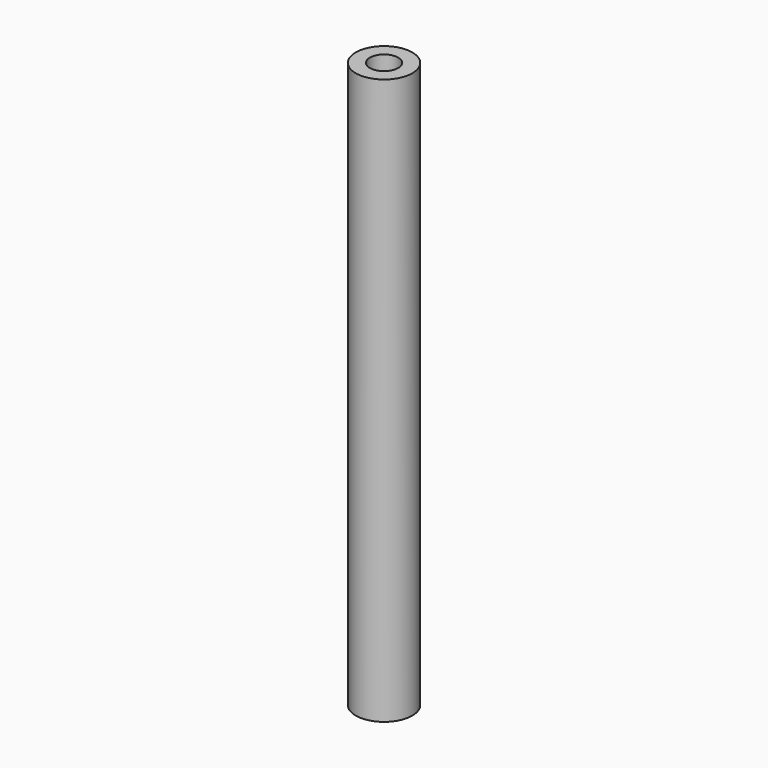
from build123d import *

# Parameters (mm, degrees)
F0_R     = 1
F0_R_2   = 0.5
F1_DEPTH = 20


# Not quite as in the source:
# - a feature names something its author has since deleted; it is built from what else it names


with BuildPart() as f1:
    # F0 (on Top) → F1 (new body)
    with BuildSketch(Plane.XY):
        Circle(F0_R)
        Circle(F0_R_2, mode=Mode.SUBTRACT)
    extrude(amount=F1_DEPTH)


solid = f1.part
